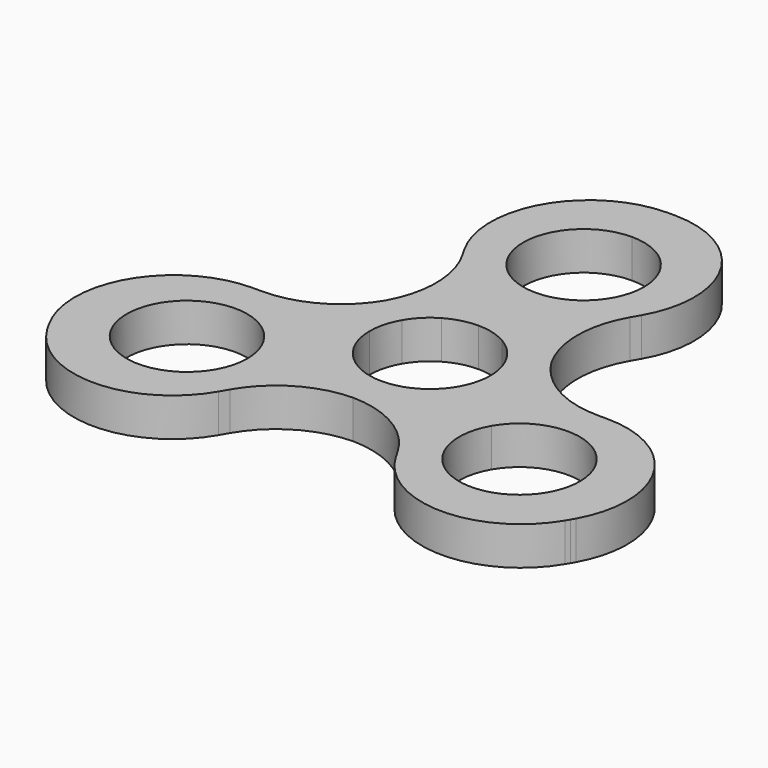
from build123d import *

# Parameters (mm, degrees)
F1_DEPTH    = 7
F2_R        = 18
F3_T1_DEPTH = 7


# Not quite as in the source:
# - a fillet or chamfer that OpenCascade refuses, or shapes differently, is made with other operations: its cross-section is extruded or revolved along the edge and cut away or added


with BuildPart() as f1:
    # F0 (on Top) → F1 (new body)
    with BuildSketch(Plane.XY):
        with BuildLine():
            ThreePointArc((9.5262794416, 5.5), (10.6251840892, 2.8470094961), (11, 0))
            Line((11, 0), (15, 0))
            ThreePointArc((15, 0), (14.4888873943, 3.8822856765), (12.9903810568, 7.5))
            Line((12.9903810568, 7.5), (9.5262794416, 5.5))
        make_face()
        with BuildLine():
            ThreePointArc((5.5, 9.5262794416), (7.7781745931, 7.7781745931), (9.5262794416, 5.5))
            Line((9.5262794416, 5.5), (12.9903810568, 7.5))
            ThreePointArc((12.9903810568, 7.5), (10.6066017178, 10.6066017178), (7.5, 12.9903810568))
            Line((7.5, 12.9903810568), (5.5, 9.5262794416))
        make_face()
        with BuildLine():
            ThreePointArc((0, 11), (2.8470094961, 10.6251840892), (5.5, 9.5262794416))
            Line((5.5, 9.5262794416), (7.5, 12.9903810568))
            ThreePointArc((7.5, 12.9903810568), (3.8822856765, 14.4888873943), (0, 15))
            Line((0, 15), (0, 11))
        make_face()
        with BuildLine():
            ThreePointArc((-5.5, 9.5262794416), (-2.8470094961, 10.6251840892), (0, 11))
            Line((0, 11), (0, 15))
            ThreePointArc((0, 15), (-3.8822856765, 14.4888873943), (-7.5, 12.9903810568))
            Line((-7.5, 12.9903810568), (-5.5, 9.5262794416))
        make_face()
        with BuildLine():
            ThreePointArc((-9.5262794416, 5.5), (-7.7781745931, 7.7781745931), (-5.5, 9.5262794416))
            Line((-5.5, 9.5262794416), (-7.5, 12.9903810568))
            ThreePointArc((-7.5, 12.9903810568), (-10.6066017178, 10.6066017178), (-12.9903810568, 7.5))
            Line((-12.9903810568, 7.5), (-9.5262794416, 5.5))
        make_face()
        with BuildLine():
            ThreePointArc((-11, 0), (-10.6251840892, 2.8470094961), (-9.5262794416, 5.5))
            Line((-9.5262794416, 5.5), (-12.9903810568, 7.5))
            ThreePointArc((-12.9903810568, 7.5), (-14.4888873943, 3.8822856765), (-15, 0))
            Line((-15, 0), (-11, 0))
        make_face()
        with BuildLine():
            Line((-12.9903810568, -7.5), (-9.5262794416, -5.5))
            ThreePointArc((-9.5262794416, -5.5), (-10.6251840892, -2.8470094961), (-11, 0))
            Line((-11, 0), (-15, 0))
            ThreePointArc((-15, 0), (-14.4888873943, -3.8822856765), (-12.9903810568, -7.5))
        make_face()
        with BuildLine():
            Line((-7.5, -12.9903810568), (-5.5, -9.5262794416))
            ThreePointArc((-5.5, -9.5262794416), (-7.7781745931, -7.7781745931), (-9.5262794416, -5.5))
            Line((-9.5262794416, -5.5), (-12.9903810568, -7.5))
            ThreePointArc((-12.9903810568, -7.5), (-10.6066017178, -10.6066017178), (-7.5, -12.9903810568))
        make_face()
        with BuildLine():
            Line((0, -15), (0, -11))
            ThreePointArc((0, -11), (-2.8470094961, -10.6251840892), (-5.5, -9.5262794416))
            Line((-5.5, -9.5262794416), (-7.5, -12.9903810568))
            ThreePointArc((-7.5, -12.9903810568), (-3.8822856765, -14.4888873943), (0, -15))
        make_face()
        with BuildLine():
            Line((7.5, -12.9903810568), (5.5, -9.5262794416))
            ThreePointArc((5.5, -9.5262794416), (2.8470094961, -10.6251840892), (0, -11))
            Line((0, -11), (0, -15))
            ThreePointArc((0, -15), (3.8822856765, -14.4888873943), (7.5, -12.9903810568))
        make_face()
        with BuildLine():
            Line((12.9903810568, -7.5), (9.5262794416, -5.5))
            ThreePointArc((9.5262794416, -5.5), (7.7781745931, -7.7781745931), (5.5, -9.5262794416))
            Line((5.5, -9.5262794416), (7.5, -12.9903810568))
            ThreePointArc((7.5, -12.9903810568), (10.6066017178, -10.6066017178), (12.9903810568, -7.5))
        make_face()
        with BuildLine():
            Line((15, 0), (11, 0))
            ThreePointArc((11, 0), (10.6251840892, -2.8470094961), (9.5262794416, -5.5))
            Line((9.5262794416, -5.5), (12.9903810568, -7.5))
            ThreePointArc((12.9903810568, -7.5), (14.4888873943, -3.8822856765), (15, 0))
        make_face()
        with BuildLine():
            Line((-8.75, -15.1554445662), (-7.5, -12.9903810568))
            ThreePointArc((-7.5, -12.9903810568), (-10.6066017178, -10.6066017178), (-12.9903810568, -7.5))
            Line((-12.9903810568, -7.5), (-15.1554445662, -8.75))
            ThreePointArc((-15.1554445662, -8.75), (-12.3743686708, -12.3743686708), (-8.75, -15.1554445662))
        make_face()
        with BuildLine():
            ThreePointArc((-7.5, 12.9903810568), (-3.8822856765, 14.4888873943), (0, 15))
            Line((0, 15), (0, 17.5))
            ThreePointArc((0, 17.5), (-4.5293332893, 16.9037019601), (-8.75, 15.1554445662))
            Line((-8.75, 15.1554445662), (-7.5, 12.9903810568))
        make_face()
        with BuildLine():
            ThreePointArc((0, 15), (3.8822856765, 14.4888873943), (7.5, 12.9903810568))
            Line((7.5, 12.9903810568), (8.75, 15.1554445662))
            ThreePointArc((8.75, 15.1554445662), (4.5293332893, 16.9037019601), (0, 17.5))
            Line((0, 17.5), (0, 15))
        make_face()
        with BuildLine():
            Line((-15.1554445662, -8.75), (-12.9903810568, -7.5))
            ThreePointArc((-12.9903810568, -7.5), (-14.4888873943, -3.8822856765), (-15, 0))
            Line((-15, 0), (-17.5, 0))
            ThreePointArc((-17.5, 0), (-16.9037019601, -4.5293332893), (-15.1554445662, -8.75))
        make_face()
        with BuildLine():
            Line((17.5, 0), (15, 0))
            ThreePointArc((15, 0), (14.4888873943, -3.8822856765), (12.9903810568, -7.5))
            Line((12.9903810568, -7.5), (15.1554445662, -8.75))
            ThreePointArc((15.1554445662, -8.75), (16.9037019601, -4.5293332893), (17.5, 0))
        make_face()
        with BuildLine():
            Line((15.1554445662, -8.75), (12.9903810568, -7.5))
            ThreePointArc((12.9903810568, -7.5), (10.6066017178, -10.6066017178), (7.5, -12.9903810568))
            Line((7.5, -12.9903810568), (8.75, -15.1554445662))
            ThreePointArc((8.75, -15.1554445662), (12.3743686708, -12.3743686708), (15.1554445662, -8.75))
        make_face()
        with BuildLine():
            Line((-20.7846096908, -12), (-17.3205080757, -10))
            ThreePointArc((-17.3205080757, -10), (-37.8108891325, -4.5096189432), (-43.3012701892, -25))
            Line((-43.3012701892, -25), (-39.8371685741, -23))
            ThreePointArc((-39.8371685741, -23), (-35.8108891325, -7.9737205584), (-20.7846096908, -12))
        make_face()
        with BuildLine():
            ThreePointArc((45.3108891325, -17.5), (34.193174809, -3.0111126057), (17.3205080757, -10))
            Line((17.3205080757, -10), (20.7846096908, -12))
            ThreePointArc((20.7846096908, -12), (33.1578986286, -6.8748159108), (41.3108891325, -17.5))
            ThreePointArc((41.3108891325, -17.5), (40.9360732216, -20.3470094961), (39.8371685741, -23))
            Line((39.8371685741, -23), (43.3012701892, -25))
            ThreePointArc((43.3012701892, -25), (44.7997765268, -21.3822856765), (45.3108891325, -17.5))
        make_face()
        with BuildLine():
            Line((20.7846096908, -12), (17.3205080757, -10))
            ThreePointArc((17.3205080757, -10), (22.8108891325, -30.4903810568), (43.3012701892, -25))
            Line((43.3012701892, -25), (39.8371685741, -23))
            ThreePointArc((39.8371685741, -23), (24.8108891325, -27.0262794416), (20.7846096908, -12))
        make_face()
        with BuildLine():
            ThreePointArc((0, 50), (-15, 35), (0, 20))
            Line((0, 20), (0, 24))
            ThreePointArc((0, 24), (-11, 35), (0, 46))
            Line((0, 46), (0, 50))
        make_face()
        with BuildLine():
            Line((0, 24), (0, 20))
            ThreePointArc((0, 20), (10.6066017178, 24.3933982822), (15, 35))
            ThreePointArc((15, 35), (10.6066017178, 45.6066017178), (0, 50))
            Line((0, 50), (0, 46))
            ThreePointArc((0, 46), (7.7781745931, 42.7781745931), (11, 35))
            ThreePointArc((11, 35), (7.7781745931, 27.2218254069), (0, 24))
        make_face()
        with BuildLine():
            ThreePointArc((-15.3108891325, -17.5), (-15.8220017381, -13.6177143235), (-17.3205080757, -10))
            Line((-17.3205080757, -10), (-20.7846096908, -12))
            ThreePointArc((-20.7846096908, -12), (-19.6857050433, -14.6529905039), (-19.3108891325, -17.5))
            ThreePointArc((-19.3108891325, -17.5), (-27.4638796363, -28.1251840892), (-39.8371685741, -23))
            Line((-39.8371685741, -23), (-43.3012701892, -25))
            ThreePointArc((-43.3012701892, -25), (-26.4286034559, -31.9888873943), (-15.3108891325, -17.5))
        make_face()
        with BuildLine():
            ThreePointArc((-8.75, 15.1554445662), (-4.5293332893, 16.9037019601), (0, 17.5))
            Line((0, 17.5), (0, 20))
            ThreePointArc((0, 20), (-15, 35), (0, 50))
            Line((0, 50), (0, 55))
            ThreePointArc((0, 55), (-14.2350474806, 53.1259204459), (-27.5, 47.6313972081))
            Line((-27.5, 47.6313972081), (-8.75, 15.1554445662))
        make_face()
        with BuildLine():
            ThreePointArc((-12.9903810568, 7.5), (-10.6066017178, 10.6066017178), (-7.5, 12.9903810568))
            Line((-7.5, 12.9903810568), (-8.75, 15.1554445662))
            ThreePointArc((-8.75, 15.1554445662), (-12.3743686708, 12.3743686708), (-15.1554445662, 8.75))
            Line((-15.1554445662, 8.75), (-12.9903810568, 7.5))
        make_face()
        with BuildLine():
            Line((-17.3205080757, -10), (-15.1554445662, -8.75))
            ThreePointArc((-15.1554445662, -8.75), (-16.9037019601, -4.5293332893), (-17.5, 0))
            Line((-17.5, 0), (-55, 0))
            ThreePointArc((-55, 0), (-53.1259204459, -14.2350474806), (-47.6313972081, -27.5))
            Line((-47.6313972081, -27.5), (-43.3012701892, -25))
            ThreePointArc((-43.3012701892, -25), (-37.8108891325, -4.5096189432), (-17.3205080757, -10))
        make_face()
        with BuildLine():
            Line((-27.5, -47.6313972081), (-8.75, -15.1554445662))
            ThreePointArc((-8.75, -15.1554445662), (-12.3743686708, -12.3743686708), (-15.1554445662, -8.75))
            Line((-15.1554445662, -8.75), (-17.3205080757, -10))
            ThreePointArc((-17.3205080757, -10), (-15.8220017381, -13.6177143235), (-15.3108891325, -17.5))
            ThreePointArc((-15.3108891325, -17.5), (-26.4286034559, -31.9888873943), (-43.3012701892, -25))
            Line((-43.3012701892, -25), (-47.6313972081, -27.5))
            ThreePointArc((-47.6313972081, -27.5), (-38.8908729653, -38.8908729653), (-27.5, -47.6313972081))
        make_face()
        with BuildLine():
            Line((0, -17.5), (0, -15))
            ThreePointArc((0, -15), (-3.8822856765, -14.4888873943), (-7.5, -12.9903810568))
            Line((-7.5, -12.9903810568), (-8.75, -15.1554445662))
            ThreePointArc((-8.75, -15.1554445662), (-4.5293332893, -16.9037019601), (0, -17.5))
        make_face()
        with BuildLine():
            Line((8.75, -15.1554445662), (7.5, -12.9903810568))
            ThreePointArc((7.5, -12.9903810568), (3.8822856765, -14.4888873943), (0, -15))
            Line((0, -15), (0, -17.5))
            ThreePointArc((0, -17.5), (4.5293332893, -16.9037019601), (8.75, -15.1554445662))
        make_face()
        with BuildLine():
            Line((17.3205080757, -10), (15.1554445662, -8.75))
            ThreePointArc((15.1554445662, -8.75), (12.3743686708, -12.3743686708), (8.75, -15.1554445662))
            Line((8.75, -15.1554445662), (27.5, -47.6313972081))
            ThreePointArc((27.5, -47.6313972081), (38.8908729653, -38.8908729653), (47.6313972081, -27.5))
            Line((47.6313972081, -27.5), (43.3012701892, -25))
            ThreePointArc((43.3012701892, -25), (22.8108891325, -30.4903810568), (17.3205080757, -10))
        make_face()
        with BuildLine():
            ThreePointArc((-15, 0), (-14.4888873943, 3.8822856765), (-12.9903810568, 7.5))
            Line((-12.9903810568, 7.5), (-15.1554445662, 8.75))
            ThreePointArc((-15.1554445662, 8.75), (-16.9037019601, 4.5293332893), (-17.5, 0))
            Line((-17.5, 0), (-15, 0))
        make_face()
        with BuildLine():
            ThreePointArc((0, 17.5), (4.5293332893, 16.9037019601), (8.75, 15.1554445662))
            Line((8.75, 15.1554445662), (27.5, 47.6313972081))
            ThreePointArc((27.5, 47.6313972081), (14.2350474806, 53.1259204459), (0, 55))
            Line((0, 55), (0, 50))
            ThreePointArc((0, 50), (10.6066017178, 45.6066017178), (15, 35))
            ThreePointArc((15, 35), (10.6066017178, 24.3933982822), (0, 20))
            Line((0, 20), (0, 17.5))
        make_face()
        with BuildLine():
            Line((55, 0), (17.5, 0))
            ThreePointArc((17.5, 0), (16.9037019601, -4.5293332893), (15.1554445662, -8.75))
            Line((15.1554445662, -8.75), (17.3205080757, -10))
            ThreePointArc((17.3205080757, -10), (34.193174809, -3.0111126057), (45.3108891325, -17.5))
            ThreePointArc((45.3108891325, -17.5), (44.7997765268, -21.3822856765), (43.3012701892, -25))
            Line((43.3012701892, -25), (47.6313972081, -27.5))
            ThreePointArc((47.6313972081, -27.5), (53.1259204459, -14.2350474806), (55, 0))
        make_face()
        with BuildLine():
            ThreePointArc((7.5, 12.9903810568), (10.6066017178, 10.6066017178), (12.9903810568, 7.5))
            Line((12.9903810568, 7.5), (15.1554445662, 8.75))
            ThreePointArc((15.1554445662, 8.75), (12.3743686708, 12.3743686708), (8.75, 15.1554445662))
            Line((8.75, 15.1554445662), (7.5, 12.9903810568))
        make_face()
        with BuildLine():
            ThreePointArc((12.9903810568, 7.5), (14.4888873943, 3.8822856765), (15, 0))
            Line((15, 0), (17.5, 0))
            ThreePointArc((17.5, 0), (16.9037019601, 4.5293332893), (15.1554445662, 8.75))
            Line((15.1554445662, 8.75), (12.9903810568, 7.5))
        make_face()
    extrude(amount=F1_DEPTH)

    # F2
    f2_edges = [f1.edges().sort_by_distance(p)[0] for p in [
        (-27.5, -47.631397, 3.5),
        (27.5, -47.631397, 3.5),
        (55, 0, 3.5),
        (27.5, 47.631397, 3.5),
        (-55, 0, 3.5),
        (-27.5, 47.631397, 3.5),
    ]]
    fillet(f2_edges, radius=F2_R)

    # F3: fillet of radius 18 on 6 edges, made by hand

    # F3_s2 → F3_t1 (join)
    with BuildSketch(Plane.XY):
        with BuildLine():
            ThreePointArc((15.0836209811, 8.8732394366), (21.6618075989, 2.3749929577), (30.5982025616, 0))
            Line((30.5982025616, 0), (17.5, 0))
            ThreePointArc((17.5, 0), (16.8851024156, 4.5981862093), (15.0836209811, 8.8732394366))
        make_face()
        with BuildLine():
            ThreePointArc((15.2991012808, 26.4988207285), (12.8877080347, 17.5721791936), (15.2262612565, 8.6261792323))
            ThreePointArc((15.2262612565, 8.6261792323), (12.4246972764, 12.3238345327), (8.75, 15.1554445662))
            Line((8.75, 15.1554445662), (15.2991012808, 26.4988207285))
        make_face()
        with BuildLine():
            ThreePointArc((0.1426402754, -17.499418669), (-8.7740995642, -19.9471721514), (-15.2991012808, -26.4988207285))
            Line((-15.2991012808, -26.4988207285), (-8.75, -15.1554445662))
            ThreePointArc((-8.75, -15.1554445662), (-4.4604051392, -16.9220207421), (0.1426402754, -17.499418669))
        make_face()
        with BuildLine():
            ThreePointArc((15.2991012808, -26.4988207285), (8.7740995642, -19.9471721514), (-0.1426402754, -17.499418669))
            ThreePointArc((-0.1426402754, -17.499418669), (4.4604051392, -16.9220207421), (8.75, -15.1554445662))
            Line((8.75, -15.1554445662), (15.2991012808, -26.4988207285))
        make_face()
        with BuildLine():
            ThreePointArc((-15.2991012808, 26.4988207285), (-12.8877080347, 17.5721791936), (-15.2262612565, 8.6261792323))
            ThreePointArc((-15.2262612565, 8.6261792323), (-12.4246972764, 12.3238345327), (-8.75, 15.1554445662))
            Line((-8.75, 15.1554445662), (-15.2991012808, 26.4988207285))
        make_face()
        with BuildLine():
            ThreePointArc((-15.0836209811, 8.8732394366), (-21.6618075989, 2.3749929577), (-30.5982025616, 0))
            Line((-30.5982025616, 0), (-17.5, 0))
            ThreePointArc((-17.5, 0), (-16.8851024156, 4.5981862093), (-15.0836209811, 8.8732394366))
        make_face()
    extrude(amount=F3_T1_DEPTH)


solid = f1.part
